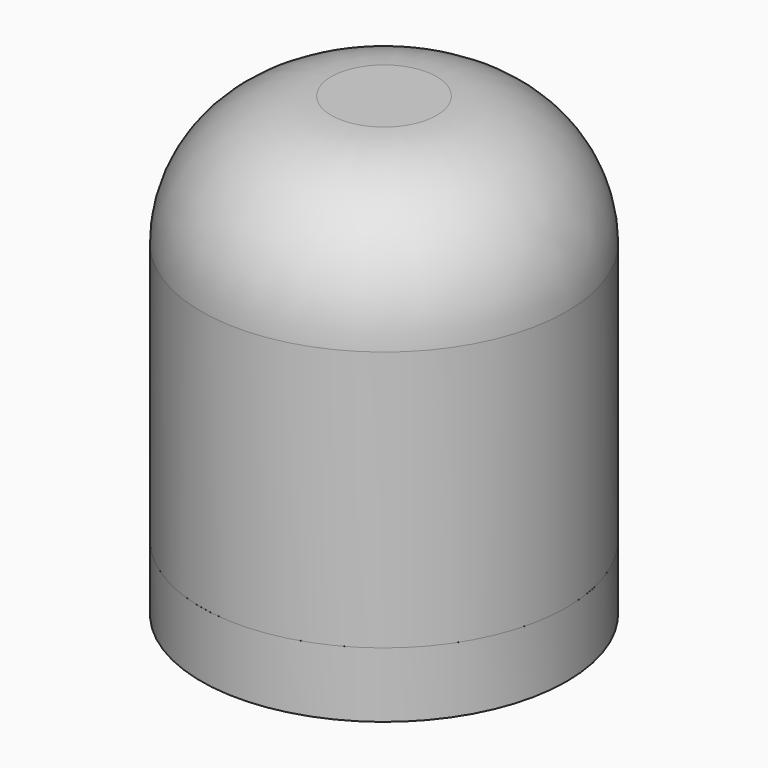
from build123d import *

# Parameters (mm, degrees)
F0_W     = 2.5650248432
F0_H     = 12.7
F2_R     = 8.9154
F2_R_2   = 8.9150248432
F2_R_3   = 6.35
F3_DEPTH = 6.35
F4_R     = 6.34999
F5_R     = 8.9154
F5_R_2   = 8.9150248432
F5_R_3   = 6.35
F6_DEPTH = 3.175


# Not quite as in the source:
# - a fillet or chamfer is up to 0.001 mm smaller than in the source, because OpenCascade refuses the exact size


with BuildPart() as f1:
    # F0 (on Front) → F1 (revolve)
    with BuildSketch(Plane.XZ):
        with Locations((-27.5444276631, -5.2465572953)):
            Rectangle(F0_W, F0_H)
    revolve(axis=Axis((-19.9119152415, 0, -5.2465572953), (0, 0, -1)))

    # F5 (on face) → F6 (join)
    with BuildSketch(Plane(origin=(0, 0, -11.5965572953), x_dir=(1, 0, 0), z_dir=(0, 0, -1))):
        with Locations((-19.9119152415, 0)):
            Circle(F5_R)
        with Locations((-19.9119152415, 0)):
            Circle(F5_R_2, mode=Mode.SUBTRACT)
        with Locations((-19.9119152415, 0)):
            Circle(F5_R_2)
        with Locations((-19.9119152415, 0)):
            Circle(F5_R_3, mode=Mode.SUBTRACT)
    extrude(amount=F6_DEPTH)


with BuildPart() as f3:
    # F2 (on face) → F3 (new body)
    with BuildSketch(Plane.XY.offset(1.1034427047)):
        with Locations((-19.9119152415, 0)):
            Circle(F2_R)
        with Locations((-19.9119152415, 0)):
            Circle(F2_R_2, mode=Mode.SUBTRACT)
        with Locations((-19.9119152415, 0)):
            Circle(F2_R_2)
        with Locations((-19.9119152415, 0)):
            Circle(F2_R_3, mode=Mode.SUBTRACT)
        with Locations((-19.9119152415, 0)):
            Circle(F2_R_3)
    extrude(amount=F3_DEPTH)

    # F4 (radius 6.35 in the source; OpenCascade refuses exactly that, so slightly less here)
    f4_edges = [f3.edges().sort_by_distance(p)[0] for p in [
        (-28.827315, 0, 7.453443),
    ]]
    fillet(f4_edges, radius=F4_R)


solid = Compound([f1.part, f3.part])
